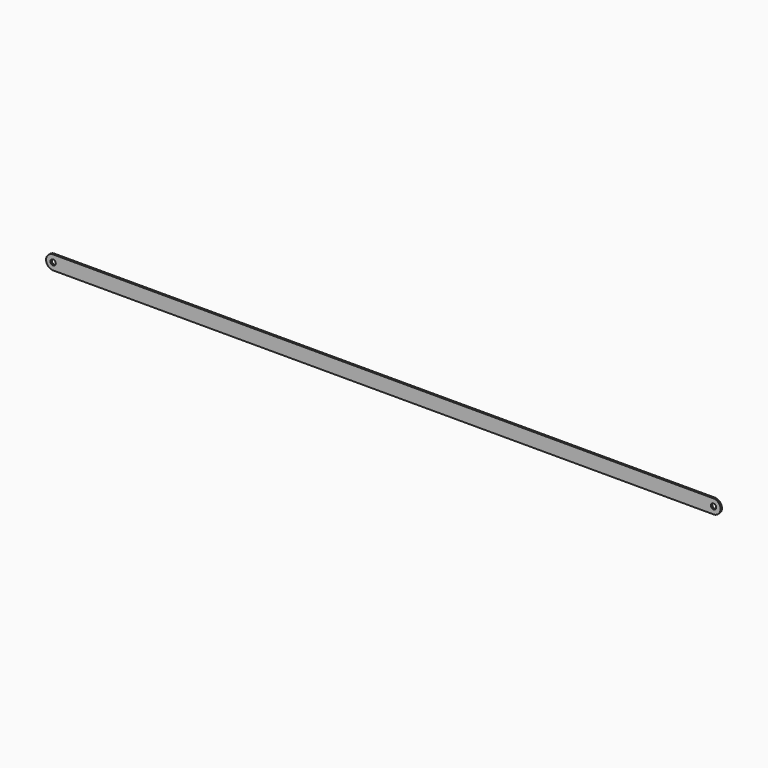
from build123d import *

# Parameters (mm, degrees)
F0_W     = 1219.2
F0_H     = 25.4
F1_DEPTH = 3.175
F2_R     = 12.69999
F3_R     = 4.8006
F4_DEPTH = 3.175


# Not quite as in the source:
# - a fillet or chamfer is up to 0.001 mm smaller than in the source, because OpenCascade refuses the exact size


with BuildPart() as f1:
    # F0 (on Front) → F1 (new body)
    with BuildSketch(Plane.XZ):
        with Locations((-73.2265757293, 35.5002675663)):
            Rectangle(F0_W, F0_H)
    extrude(amount=F1_DEPTH)

    # F2 (radius 12.7 in the source; OpenCascade refuses exactly that, so slightly less here)
    f2_edges = [f1.edges().sort_by_distance(p)[0] for p in [
        (536.373424, -1.5875, 48.200268),
        (536.373424, -1.5875, 22.800268),
        (-682.826576, -1.5875, 48.200268),
        (-682.826576, -1.5875, 22.800268),
    ]]
    fillet(f2_edges, radius=F2_R)

    # F3 (on face) → F4 (cut)
    with BuildSketch(Plane.XZ.offset(3.175)):
        with Locations((-670.1265757293, 35.5002675663)):
            Circle(F3_R)
        with Locations((523.6734242707, 35.5002675663)):
            Circle(F3_R)
    extrude(amount=-F4_DEPTH, mode=Mode.SUBTRACT)


solid = f1.part
